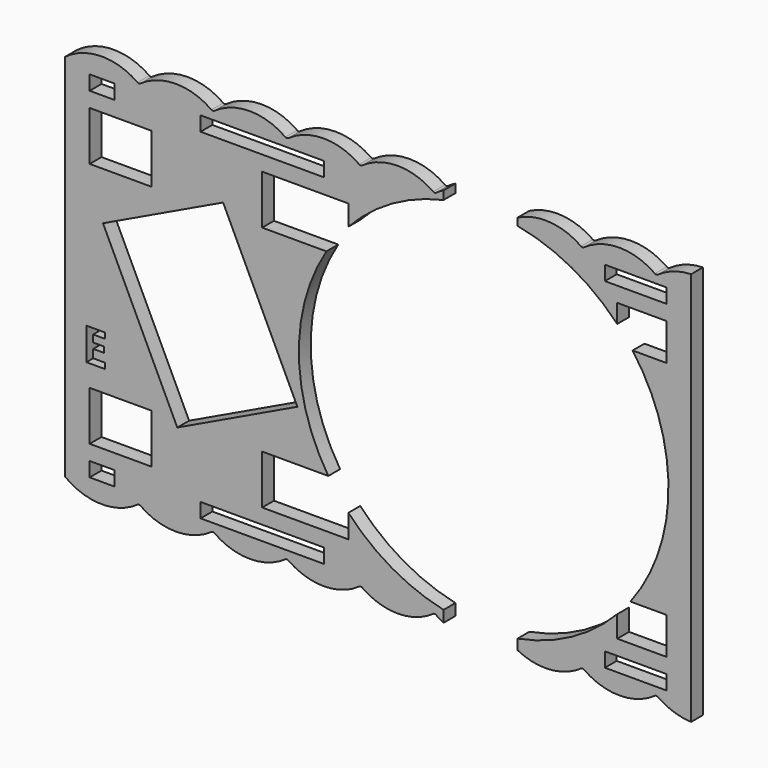
from build123d import *

# Parameters (mm, degrees)
F0_W         = 254.1
F0_H         = 160
F0_R         = 75
F2_DEPTH     = 6
F3_W         = 30
F3_H         = 20
F4_DEPTH     = 25
F5_W         = 10
F5_H         = 5.87
F5_W_2       = 50
F5_W_3       = 25
F6_DEPTH     = 11
F7_W         = 25
F7_H         = 20
F7_W_2       = 35
F7_W_3       = 20
F7_H_2       = 15
F8_DEPTH     = 25
F9_TEXT_SIZE = 18.3131300016
F10_DEPTH    = 25


# Not quite as in the source:
# - Text() gives the source's letters only with a copy of the font that has no kerning and outlines rounded to 1/6400 em; it was checked with that copy


with BuildPart() as f2:
    # F0 (on Front) → F2 (new body)
    with BuildSketch(Plane.XZ):
        with Locations((-13.9171167456, 18.0924118194)):
            Rectangle(F0_W, F0_H)
        Polygon((-125.5614100839, 38.6465899695), (-76.8291792837, 61.9096439659), (-46.6733685477, -1.2617663307), (-95.4055993479, -24.524820327), align=None, mode=Mode.SUBTRACT)
        with Locations((28.9328832544, 18.6924118194)):
            Circle(F0_R, mode=Mode.SUBTRACT)
    extrude(amount=-F2_DEPTH)

    # F3 (on face) → F4 (cut)
    with BuildSketch(Plane.XZ):
        with Locations((27.6538580656, 98.0924118194)):
            Rectangle(F3_W, F3_H)
        with Locations((27.6538580656, -61.9075881806)):
            Rectangle(F3_W, F3_H)
    extrude(amount=-F4_DEPTH, mode=Mode.SUBTRACT)

    # F5 (on Front) → F6 (cut)
    with BuildSketch(Plane.XZ):
        with Locations((-125.9671167456, 87.1574118194)):
            Rectangle(F5_W, F5_H)
        with Locations((-60.9671167456, 87.1574118194)):
            Rectangle(F5_W_2, F5_H)
        with Locations((90.6328832544, 87.1574118194)):
            Rectangle(F5_W_3, F5_H)
        with Locations((90.6328832544, -50.9725881806)):
            Rectangle(F5_W_3, F5_H)
        with Locations((-125.9671167456, -50.9725881806)):
            Rectangle(F5_W, F5_H)
        with Locations((-60.9671167456, -50.9725881806)):
            Rectangle(F5_W_2, F5_H)
    extrude(amount=-F6_DEPTH, mode=Mode.SUBTRACT)

    # F7 (on Front) → F8 (cut)
    with BuildSketch(Plane.XZ):
        with BuildLine():
            ThreePointArc((-140.9671167456, 93.0924118194), (-126.3239109441, 98.0898656478), (-111.5440398226, 93.5123739171))
            ThreePointArc((-111.5440398226, 93.5123739171), (-110.9671167456, 93.329172401), (-110.3901936687, 93.5123739171))
            ThreePointArc((-110.3901936687, 93.5123739171), (-95.9671167456, 98.0924118194), (-81.5440398226, 93.5123739171))
            ThreePointArc((-81.5440398226, 93.5123739171), (-80.9671167456, 93.329172401), (-80.3901936687, 93.5123739171))
            ThreePointArc((-80.3901936687, 93.5123739171), (-65.9671167456, 98.0924118194), (-51.5440398226, 93.5123739171))
            ThreePointArc((-51.5440398226, 93.5123739171), (-50.9671167456, 93.329172401), (-50.3901936687, 93.5123739171))
            ThreePointArc((-50.3901936687, 93.5123739171), (-35.9671167456, 98.0924118194), (-21.5440398226, 93.5123739171))
            ThreePointArc((-21.5440398226, 93.5123739171), (-20.9671167456, 93.329172401), (-20.3901936687, 93.5123739171))
            ThreePointArc((-20.3901936687, 93.5123739171), (-5.9671167456, 98.0924118194), (8.4559601774, 93.5123739171))
            ThreePointArc((8.4559601774, 93.5123739171), (9.0328832544, 93.329172401), (9.6098063313, 93.5123739171))
            ThreePointArc((9.6098063313, 93.5123739171), (24.0328832544, 98.0924118194), (38.4559601774, 93.5123739171))
            ThreePointArc((38.4559601774, 93.5123739171), (39.0328832544, 93.329172401), (39.6098063313, 93.5123739171))
            ThreePointArc((39.6098063313, 93.5123739171), (54.0328832544, 98.0924118194), (68.4559601774, 93.5123739171))
            ThreePointArc((68.4559601774, 93.5123739171), (69.0328832544, 93.329172401), (69.6098063313, 93.5123739171))
            ThreePointArc((69.6098063313, 93.5123739171), (84.0328832544, 98.0924118194), (98.4559601774, 93.5123739171))
            ThreePointArc((98.4559601774, 93.5123739171), (99.0328832544, 93.329172401), (99.6098063313, 93.5123739171))
            ThreePointArc((99.6098063313, 93.5123739171), (114.3896774528, 98.0898656478), (129.0328832544, 93.0924118194))
            ThreePointArc((129.0328832544, 93.0924118194), (144.0328832544, 98.0924118194), (159.0328832544, 93.0924118194))
            Line((159.0328832544, 93.0924118194), (159.0010523796, 104.872263968))
            Line((159.0010523796, 104.872263968), (-149.2778658867, 104.872263968))
            Line((-149.2778658867, 104.872263968), (-149.2778658867, 93.0924118194))
            Line((-149.2778658867, 93.0924118194), (-140.9671167456, 93.0924118194))
        make_face()
        with BuildLine():
            ThreePointArc((69.6098063313, -57.3275502783), (69.0328832544, -57.1443487622), (68.4559601774, -57.3275502783))
            ThreePointArc((68.4559601774, -57.3275502783), (54.0328832544, -61.9075881806), (39.6098063313, -57.3275502783))
            ThreePointArc((39.6098063313, -57.3275502783), (39.0328832544, -57.1443487622), (38.4559601774, -57.3275502783))
            ThreePointArc((38.4559601774, -57.3275502783), (24.0328832544, -61.9075881806), (9.6098063313, -57.3275502783))
            ThreePointArc((9.6098063313, -57.3275502783), (9.0328832544, -57.1443487622), (8.4559601774, -57.3275502783))
            ThreePointArc((8.4559601774, -57.3275502783), (-5.9671167456, -61.9075881806), (-20.3901936687, -57.3275502783))
            ThreePointArc((-20.3901936687, -57.3275502783), (-20.9671167456, -57.1443487622), (-21.5440398226, -57.3275502783))
            ThreePointArc((-21.5440398226, -57.3275502783), (-35.9671167456, -61.9075881806), (-50.3901936687, -57.3275502783))
            ThreePointArc((-50.3901936687, -57.3275502783), (-50.9671167456, -57.1443487622), (-51.5440398226, -57.3275502783))
            ThreePointArc((-51.5440398226, -57.3275502783), (-65.9671167456, -61.9075881806), (-80.3901936687, -57.3275502783))
            ThreePointArc((-80.3901936687, -57.3275502783), (-80.9671167456, -57.1443487622), (-81.5440398226, -57.3275502783))
            ThreePointArc((-81.5440398226, -57.3275502783), (-95.9671167456, -61.9075881806), (-110.3901936687, -57.3275502783))
            ThreePointArc((-110.3901936687, -57.3275502783), (-110.9671167456, -57.1443487622), (-111.5440398226, -57.3275502783))
            ThreePointArc((-111.5440398226, -57.3275502783), (-126.3239109441, -61.9050420089), (-140.9671167456, -56.9075881806))
            Line((-140.9671167456, -56.9075881806), (-149.2778658867, -56.9075881806))
            Line((-149.2778658867, -56.9075881806), (-149.2778658867, -68.6874403291))
            Line((-149.2778658867, -68.6874403291), (159.0010523796, -68.6874403291))
            Line((159.0010523796, -68.6874403291), (159.0328832544, -56.9075881806))
            ThreePointArc((159.0328832544, -56.9075881806), (144.0328832544, -61.9075881806), (129.0328832544, -56.9075881806))
            ThreePointArc((129.0328832544, -56.9075881806), (114.3896774528, -61.9050420089), (99.6098063313, -57.3275502783))
            ThreePointArc((99.6098063313, -57.3275502783), (99.0328832544, -57.1443487622), (98.4559601774, -57.3275502783))
            ThreePointArc((98.4559601774, -57.3275502783), (84.0328832544, -61.9075881806), (69.6098063313, -57.3275502783))
        make_face()
        with Locations((-118.4671167456, 68.0924118194)):
            Rectangle(F7_W, F7_H)
        with Locations((-43.4671167456, 68.0924118194)):
            Rectangle(F7_W_2, F7_H)
        with Locations((93.1328832544, 70.5924118194)):
            Rectangle(F7_W_3, F7_H_2)
        with Locations((93.1328832544, -34.4075881806)):
            Rectangle(F7_W_3, F7_H_2)
        with Locations((-43.4671167456, -31.9075881806)):
            Rectangle(F7_W_2, F7_H)
        with Locations((-118.4671167456, -31.9075881806)):
            Rectangle(F7_W, F7_H)
    extrude(amount=-F8_DEPTH, mode=Mode.SUBTRACT)

    # F9 (on face) → F10 (cut)
    with BuildSketch(Plane.XZ):
        with Locations((-133.9481472969, -13.1854536012)):
            Text('E', F9_TEXT_SIZE, font='Open Sans', font_style=FontStyle.BOLD, text_align=(TextAlign.LEFT, TextAlign.BOTTOM))
    extrude(amount=-F10_DEPTH, mode=Mode.SUBTRACT)


solid = f2.part
